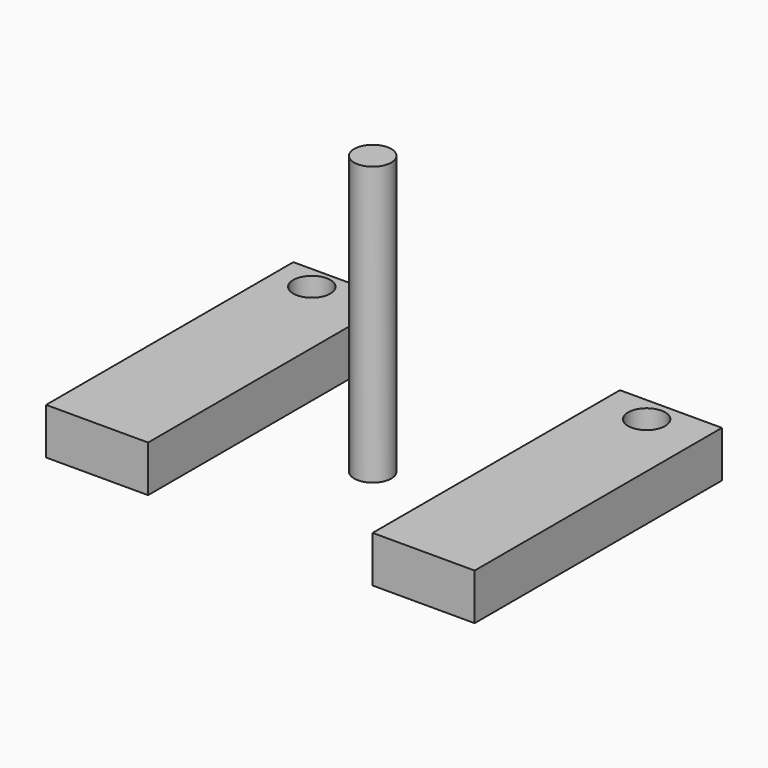
from build123d import *

# Parameters (mm, degrees)
F0_W     = 33
F0_H     = 100
F0_R     = 6
F1_DEPTH = 15
F3_DEPTH = 75


# Not quite as in the source:
# - the program builds the solid bodies; features that only make, move or delete a surface that nothing else refers to are left out


with BuildPart() as f1:
    # F0 (on Top) → F1 (new body)
    with BuildSketch(Plane.XY):
        with Locations((-52.8000037262, 4.5173896843)):
            Rectangle(F0_W, F0_H)
        with Locations((-57.2336092591, 46.9057410955)):
            Circle(F0_R, mode=Mode.SUBTRACT)
    extrude(amount=F1_DEPTH)


with BuildPart() as f1b:
    # F0 (on Top) → F1, piece 2 (new body)
    with BuildSketch(Plane.XY):
        with Locations((55.3826065895, 1.3608676211)):
            Rectangle(F0_W, F0_H)
        with Locations((54.0778711438, 43.1762300432)):
            Circle(F0_R, mode=Mode.SUBTRACT)
    extrude(amount=F1_DEPTH)


with BuildPart() as f1c:
    # F0 (on Top) → F1, piece 3 (new body)
    with BuildSketch(Plane.XY):
        Circle(F0_R)
    extrude(amount=F1_DEPTH)

    # F3 (add): a face of the model
    f3_faces = [f1c.faces().sort_by_distance(p)[0] for p in [
        (0, 0, 15),
    ]]
    extrude(f3_faces, amount=F3_DEPTH)


solid = Compound([f1.part, f1b.part, f1c.part])
